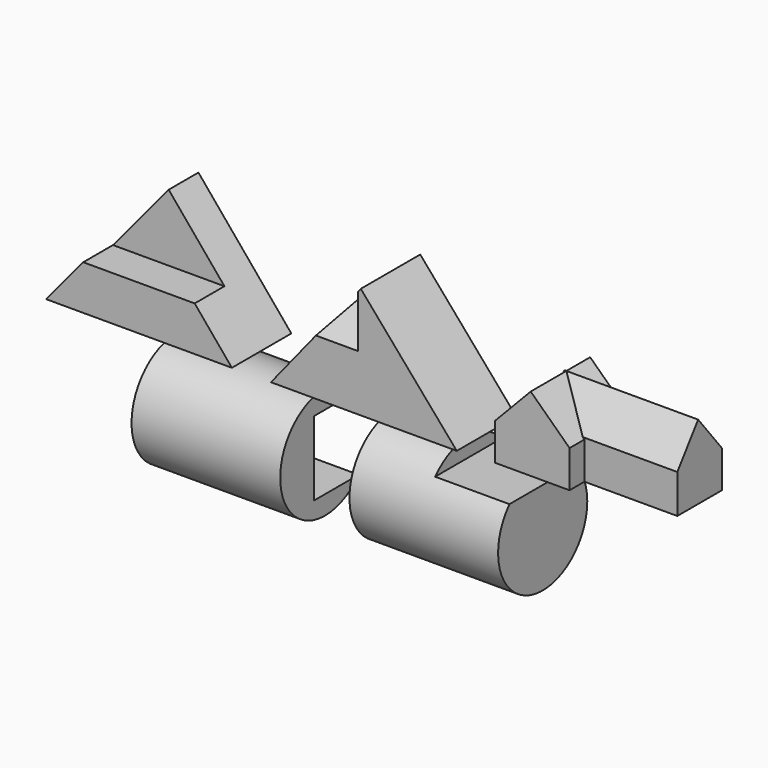
from build123d import *

# Parameters (mm, degrees)
F1_DEPTH  = 101.6
F3_DEPTH  = 50.8
F5_DEPTH  = 101.6
F8_DEPTH  = 220.98
F10_DEPTH = 101.6
F13_DEPTH = 182.88
F16_R     = 76.2
F17_DEPTH = 203.2
F20_DEPTH = 101.6
F21_R     = 76.6724448951
F22_DEPTH = 203.2
F24_DEPTH = 261.62


# Not quite as in the source:
# - a feature of the source that left no trace in its solid (it failed there, or was rolled back) is left out


with BuildPart() as f1:
    # F0 (on Front) → F1 (new body)
    with BuildSketch(Plane.XZ):
        Polygon((0, 0), (-127, -152.4), (127, -152.4), align=None)
    extrude(amount=-F1_DEPTH)

    # F2 (on face) → F3 (cut)
    with BuildSketch(Plane.XZ):
        Polygon((76.2, -91.44), (0, 0), (-76.2, -91.44), align=None)
    extrude(amount=-F3_DEPTH, mode=Mode.SUBTRACT)


with BuildPart() as f5:
    # F4 (on Front) → F5 (new body)
    with BuildSketch(Plane.XZ):
        Polygon((303.2561838627, 0), (180.4631147786, -152.4), (434.4631147786, -152.4), align=None)
    extrude(amount=-F5_DEPTH)

    # F7 (on offset) → F8 (cut)
    with BuildSketch(Plane.YZ.offset(299.72)):
        Polygon((50.8, 0), (0, 0), (0, -76.2), align=None)
    extrude(amount=-F8_DEPTH, mode=Mode.SUBTRACT)


with BuildPart() as f10:
    # F9 (on Front) → F10 (new body)
    with BuildSketch(Plane.XZ):
        Polygon((487.0548210189, -98.9035038978), (487.0548210189, -149.7035038978), (588.6548210189, -149.7035038978), (588.6548210189, -98.9035038978), (535.5460643768, -48.1035038978), align=None)
    extrude(amount=-F10_DEPTH)

    # F12 (on offset) → F13 (join)
    with BuildSketch(Plane.YZ.offset(715.6548210189)):
        Polygon((25.4286060488, -149.7035038978), (101.6286060488, -149.7035038978), (101.6286060488, -98.9035038978), (60.9574409105, -48.1035038978), (25.4286060488, -96.7219075692), align=None)
    extrude(amount=-F13_DEPTH)


with BuildPart() as f17:
    # F16 (on offset) → F17 (new body)
    with BuildSketch(Plane.YZ.offset(299.72)):
        with Locations((61.2636841834, -246.9049543142)):
            Circle(F16_R)
    extrude(amount=F17_DEPTH)

    # F19 (on face) → F20 (cut)
    with BuildSketch(Plane.YZ.offset(502.92)):
        with BuildLine():
            ThreePointArc((118.0598108119, -196.1049543142), (61.2636841834, -170.7049543142), (4.4675575549, -196.1049543142))
            Line((4.4675575549, -196.1049543142), (118.0598108119, -196.1049543142))
        make_face()
    extrude(amount=-F20_DEPTH, mode=Mode.SUBTRACT)


with BuildPart() as f22:
    # F21 (on Right) → F22 (new body)
    with BuildSketch(Plane.YZ):
        with Locations((64.0127211809, -254.9076080322)):
            Circle(F21_R)
    extrude(amount=F22_DEPTH)

    # F23 (on face) → F24 (cut)
    with BuildSketch(Plane(origin=(0, 0, 0), x_dir=(0, -1, 0), z_dir=(-1, 0, 0))):
        with BuildLine():
            Line((-45.2411445111, -204.1076080322), (-121.4411445111, -204.1076080322))
            ThreePointArc((-121.4411445111, -204.1076080322), (-140.685166076, -254.9076080322), (-121.4411445111, -305.7076080322))
            Line((-121.4411445111, -305.7076080322), (-45.2411445111, -305.7076080322))
            Line((-45.2411445111, -305.7076080322), (-45.2411445111, -204.1076080322))
        make_face()
    extrude(amount=-F24_DEPTH, mode=Mode.SUBTRACT)


solid = Compound([f1.part, f5.part, f10.part, f17.part, f22.part])
